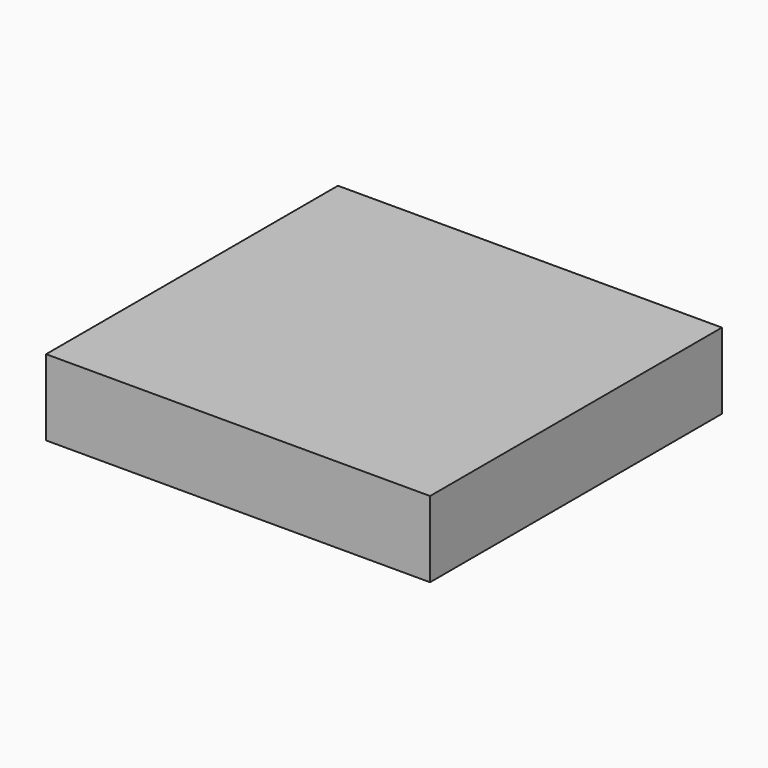
from build123d import *

# Parameters (mm, degrees)
F0_W     = 128.4354180098
F0_H     = 122.0201179385
F1_DEPTH = 25.4


# Not quite as in the source:
# - the program builds the solid bodies; features that only make, move or delete a surface that nothing else refers to are left out


with BuildPart() as f1:
    # F0 (on Top) → F1 (new body)
    with BuildSketch(Plane.XY):
        with Locations((-0.928722322, 2.4145655334)):
            Rectangle(F0_W, F0_H)
    extrude(amount=F1_DEPTH)


solid = f1.part
